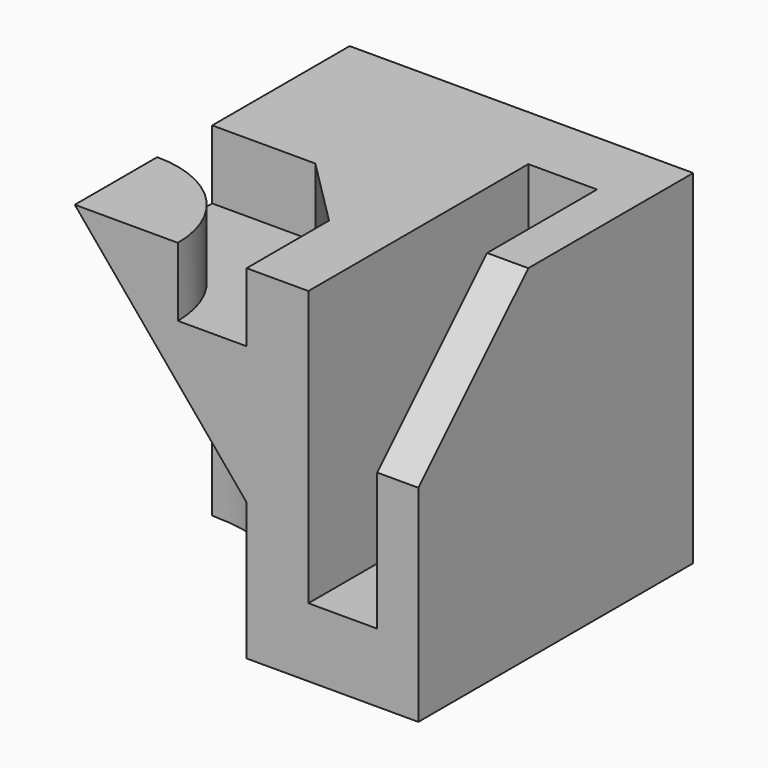
from build123d import *

# Parameters (mm, degrees)
F0_W      = 50
F0_H      = 50
F1_DEPTH  = 50
F3_DEPTH  = 6
F4_W      = 10
F4_H      = 40
F5_DEPTH  = 40
F6_R      = 10
F8_DEPTH  = 10
F9_SIZE   = 10
F11_DEPTH = 20
F12_DEPTH = 20


# Not quite as in the source:
# - a feature names something its author has since deleted; it is built from what else it names


with BuildPart() as f1:
    # F0 (on Top) → F1 (new body)
    with BuildSketch(Plane.XY):
        with Locations((25, -25)):
            Rectangle(F0_W, F0_H)
    extrude(amount=F1_DEPTH)

    # F2 (on face) → F3 (cut)
    with BuildSketch(Plane.YZ.offset(50)):
        Polygon((-30, 50), (-50, 50), (-50, 30), align=None)
    extrude(amount=-F3_DEPTH, mode=Mode.SUBTRACT)

    # F4 (on face) → F5 (cut)
    with BuildSketch(Plane.XZ.offset(50)):
        with Locations((39, 30)):
            Rectangle(F4_W, F4_H)
    extrude(amount=-F5_DEPTH, mode=Mode.SUBTRACT)

    # F6
    f6_edges = [f1.edges().sort_by_distance(p)[0] for p in [
        (39, -10, 10),
    ]]
    fillet(f6_edges, radius=F6_R)

    # F7 (on face) → F8 (cut)
    with BuildSketch(Plane.XY.offset(50)):
        with BuildLine():
            Line((0, -25), (0, -35))
            ThreePointArc((0, -35), (10.6066017178, -39.3933982822), (15, -50))
            Line((15, -50), (25, -50))
            Line((25, -50), (25, -25))
            Line((25, -25), (0, -25))
        make_face()
    extrude(amount=-F8_DEPTH, mode=Mode.SUBTRACT)

    # F9
    f9_edges = [f1.edges().sort_by_distance(p)[0] for p in [
        (25, -25, 45),
    ]]
    chamfer(f9_edges, length=F9_SIZE)

    # F10 (on face) → F11 (cut)
    with BuildSketch(Plane(origin=(0, 0, 0), x_dir=(1, 0, 0), z_dir=(0, 0, -1))):
        with BuildLine():
            Line((25, 50), (0, 50))
            Line((0, 50), (0, 25))
            ThreePointArc((0, 25), (17.6776695297, 32.3223304703), (25, 50))
        make_face()
    extrude(amount=-F11_DEPTH, mode=Mode.SUBTRACT)

    # F10 (on face) → F12 (cut)
    with BuildSketch(Plane(origin=(0, 0, 0), x_dir=(1, 0, 0), z_dir=(0, 0, -1))):
        with BuildLine():
            Line((25, 50), (0, 50))
            Line((0, 50), (0, 25))
            ThreePointArc((0, 25), (17.6776695297, 32.3223304703), (25, 50))
        make_face()
    extrude(amount=-F12_DEPTH, mode=Mode.SUBTRACT)

    # F11_face (on face) → F14 section 0
    with BuildSketch(Plane(origin=(10.6103295395, -39.3896704605, 20), x_dir=(1, 0, 0), z_dir=(0, 0, -1)), mode=Mode.PRIVATE) as f14_s0:
        with BuildLine():
            Line((14.3896704605, 10.6103295395), (-10.6103295395, 10.6103295395))
            Line((-10.6103295395, 10.6103295395), (-10.6103295395, -14.3896704605))
            ThreePointArc((-10.6103295395, -14.3896704605), (7.0673399902, -7.0673399902), (14.3896704605, 10.6103295395))
        make_face()
    loft([f14_s0.sketch, Vertex(0, -50, 50)], mode=Mode.SUBTRACT)


solid = f1.part
